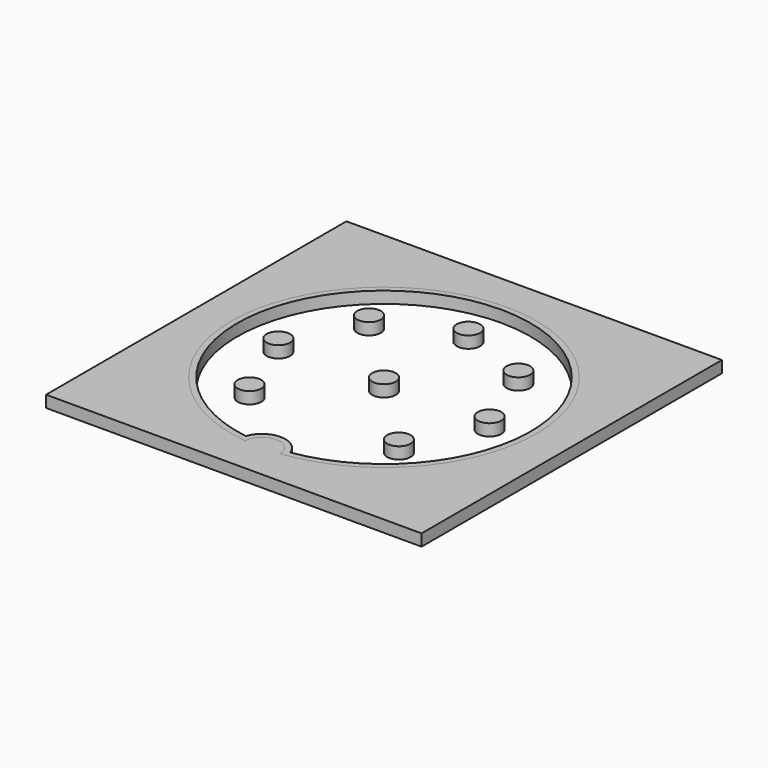
from build123d import *

# Parameters (mm, degrees)
F1_DEPTH = 1
F0_R     = 1
F0_W     = 32
F0_H     = 32
F2_DEPTH = 1


# Not quite as in the source:
# - a feature names something its author has since deleted; it is built from what else it names


with BuildPart() as f1:
    # F0 (on Top) → F1 (new body)
    with BuildSketch(Plane.XY):
        with BuildLine():
            ThreePointArc((-1.5003664489, -12.9134615385), (-0.0028648313, -11.5), (1.4946367862, -12.9134615385))
            ThreePointArc((1.4946367862, -12.9134615385), (-0.0028648313, 13), (-1.5003664489, -12.9134615385))
        make_face()
        with BuildLine():
            ThreePointArc((-1.8962656648, -12.3557692308), (-0.0028648313, 12.5), (1.8905360021, -12.3557692308))
            ThreePointArc((1.8905360021, -12.3557692308), (-0.0028648313, -11), (-1.8962656648, -12.3557692308))
        make_face(mode=Mode.SUBTRACT)
    extrude(amount=F1_DEPTH)


with BuildPart() as f1b:
    # F0 (on Top) → F1, piece 2 (new body)
    with BuildSketch(Plane.XY):
        with Locations((-6.366825862, -6.3639610307)):
            Circle(F0_R)
    extrude(amount=F1_DEPTH)


with BuildPart() as f1c:
    # F0 (on Top) → F1, piece 3 (new body)
    with BuildSketch(Plane.XY):
        with Locations((-9.0028648313, 0)):
            Circle(F0_R)
    extrude(amount=F1_DEPTH)


with BuildPart() as f1d:
    # F0 (on Top) → F1, piece 4 (new body)
    with BuildSketch(Plane.XY):
        with Locations((-6.366825862, 6.3639610307)):
            Circle(F0_R)
    extrude(amount=F1_DEPTH)


with BuildPart() as f1e:
    # F0 (on Top) → F1, piece 5 (new body)
    with BuildSketch(Plane.XY):
        with Locations((-0.0028648313, 9)):
            Circle(F0_R)
    extrude(amount=F1_DEPTH)


with BuildPart() as f1f:
    # F0 (on Top) → F1, piece 6 (new body)
    with BuildSketch(Plane.XY):
        with Locations((6.3610961993, 6.3639610307)):
            Circle(F0_R)
    extrude(amount=F1_DEPTH)


with BuildPart() as f1g:
    # F0 (on Top) → F1, piece 7 (new body)
    with BuildSketch(Plane.XY):
        with Locations((8.9971351687, 0)):
            Circle(F0_R)
    extrude(amount=F1_DEPTH)


with BuildPart() as f1h:
    # F0 (on Top) → F1, piece 8 (new body)
    with BuildSketch(Plane.XY):
        with Locations((6.3610961993, -6.3639610307)):
            Circle(F0_R)
    extrude(amount=F1_DEPTH)


with BuildPart() as f1i:
    # F0 (on Top) → F1, piece 9 (new body)
    with BuildSketch(Plane.XY):
        with Locations((-0.0028648313, 0)):
            Circle(F0_R)
    extrude(amount=F1_DEPTH)


with BuildPart() as f2:
    # F0 (on Top) → F2 (new body)
    with BuildSketch(Plane.XY):
        Rectangle(F0_W, F0_H)
        with BuildLine():
            ThreePointArc((-1.5003664489, -12.9134615385), (-0.0028648313, 13), (1.4946367862, -12.9134615385))
            ThreePointArc((1.4946367862, -12.9134615385), (-0.0028648313, -11.5), (-1.5003664489, -12.9134615385))
        make_face(mode=Mode.SUBTRACT)
    extrude(amount=F2_DEPTH)


solid = Compound([f1.part, f1b.part, f1c.part, f1d.part, f1e.part, f1f.part, f1g.part, f1h.part, f1i.part, f2.part])
